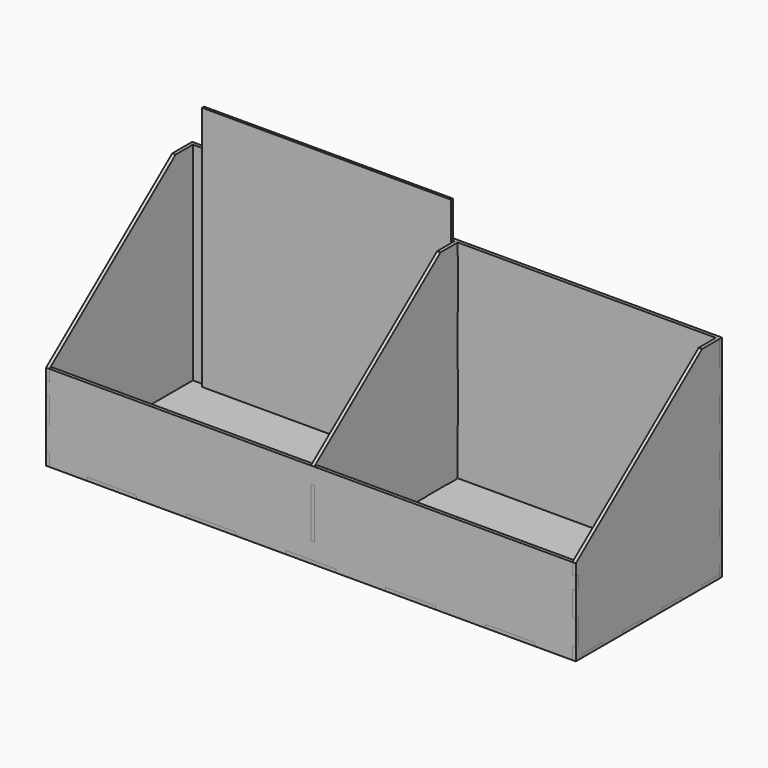
from build123d import *

# Parameters (mm, degrees)
F0_W          = 638
F0_H          = 220
F1_DEPTH      = 4
F2_W          = 638
F2_H          = 4
F3_DEPTH      = 100
F3_DEPTH_BACK = 4
F4_W          = 638
F4_H          = 4
F5_DEPTH      = 250
F5_DEPTH_BACK = 4
F7_DEPTH      = 4
F10_W         = 3
F10_H         = 300
F11_DEPTH     = 300
F12_W         = 4
F12_H         = 30
F12_W_2       = 30
F12_H_2       = 4
F12_H_3       = 15
F13_DEPTH     = 4
F15_W         = 4
F15_H         = 13.8488392308
F15_H_2       = 30
F15_H_3       = 15.1511607692
F15_W_2       = 60
F15_H_4       = 4
F15_W_3       = 4.3
F15_H_5       = 60
F16_DEPTH     = 25
F17_W         = 4
F17_H         = 20
F17_H_2       = 31.2709829547
F17_W_2       = 60
F17_H_3       = 4
F17_W_3       = 30
F17_H_4       = 60
F18_DEPTH     = 25
F19_W         = 4.3
F19_H         = 60
F19_W_2       = 4
F19_H_2       = 30
F19_W_3       = 60
F19_H_3       = 4
F20_DEPTH     = 25
F21_W         = 4.3
F21_H         = 30
F21_W_2       = 60
F21_H_2       = 4
F21_H_3       = 16
F21_W_3       = 4
F22_DEPTH     = 25


with BuildPart() as f1:
    # F0 (on Top) → F1 (new body)
    with BuildSketch(Plane.XY):
        Rectangle(F0_W, F0_H)
    extrude(amount=F1_DEPTH)

    # F21 (on face) → F22 (cut)
    with BuildSketch(Plane(origin=(0, 0, 0), x_dir=(1, 0, 0), z_dir=(0, 0, -1))):
        with Locations((2.15, 45)):
            Rectangle(F21_W, F21_H)
        with Locations((60, 108)):
            Rectangle(F21_W_2, F21_H_2)
        with Locations((180, 108)):
            Rectangle(F21_W_2, F21_H_2)
        Polygon((319, 110), (270, 110), (270, 106), (315, 106), (315, 100), (319, 100), (319, 106), align=None)
        with Locations((2.15, 98)):
            Rectangle(F21_W, F21_H_3)
        with Locations((317, 55)):
            Rectangle(F21_W_3, F21_H)
        with Locations((317, -5)):
            Rectangle(F21_W_3, F21_H)
        Polygon((319, -110), (319, -106), (315, -106), (270, -106), (270, -110), align=None)
        with Locations((2.15, -45)):
            Rectangle(F21_W, F21_H)
        with Locations((2.15, -98)):
            Rectangle(F21_W, F21_H_3)
        with Locations((60, -108)):
            Rectangle(F21_W_2, F21_H_2)
        with Locations((180, -108)):
            Rectangle(F21_W_2, F21_H_2)
        with Locations((317, -65)):
            Rectangle(F21_W_3, F21_H)
        with Locations((-180, 108)):
            Rectangle(F21_W_2, F21_H_2)
        with Locations((-317, -65)):
            Rectangle(F21_W_3, F21_H)
        Polygon((-319, 110), (-319, 106), (-319, 100), (-315, 100), (-315, 106), (-270, 106), (-270, 110), align=None)
        with Locations((-60, 108)):
            Rectangle(F21_W_2, F21_H_2)
        with Locations((-180, -108)):
            Rectangle(F21_W_2, F21_H_2)
        with Locations((-317, -5)):
            Rectangle(F21_W_3, F21_H)
        with Locations((-317, 55)):
            Rectangle(F21_W_3, F21_H)
        with Locations((-60, -108)):
            Rectangle(F21_W_2, F21_H_2)
        Polygon((-319, -110), (-270, -110), (-270, -106), (-315, -106), (-319, -106), align=None)
    extrude(amount=-F22_DEPTH, mode=Mode.SUBTRACT)


with BuildPart() as f3:
    # F2 (on face) → F3 (new body, two sides)
    with BuildSketch(Plane.XY.offset(4)) as f3_sk:
        with Locations((0, -108)):
            Rectangle(F2_W, F2_H)
    extrude(amount=F3_DEPTH)
    extrude(f3_sk.sketch, amount=-F3_DEPTH_BACK)

    # F15 (on face) → F16 (cut)
    with BuildSketch(Plane.XZ.offset(110)):
        with Locations((-317, 97.0755803846)):
            Rectangle(F15_W, F15_H)
        with Locations((-317, 60.1511607692)):
            Rectangle(F15_W, F15_H_2)
        with Locations((-317, 7.5755803846)):
            Rectangle(F15_W, F15_H_3)
        with Locations((317, 97.0755803846)):
            Rectangle(F15_W, F15_H)
        with Locations((317, 60.1511607692)):
            Rectangle(F15_W, F15_H_2)
        with Locations((317, 7.5755803846)):
            Rectangle(F15_W, F15_H_3)
        with Locations((-240, 2)):
            Rectangle(F15_W_2, F15_H_4)
        with Locations((-120, 2)):
            Rectangle(F15_W_2, F15_H_4)
        with Locations((0, 2)):
            Rectangle(F15_W_2, F15_H_4)
        with Locations((120, 2)):
            Rectangle(F15_W_2, F15_H_4)
        with Locations((240, 2)):
            Rectangle(F15_W_2, F15_H_4)
        with Locations((2.15, 54)):
            Rectangle(F15_W_3, F15_H_5)
    extrude(amount=-F16_DEPTH, mode=Mode.SUBTRACT)


with BuildPart() as f5:
    # F4 (on face) → F5 (new body, two sides)
    with BuildSketch(Plane.XY.offset(4)) as f5_sk:
        with Locations((0, 108)):
            Rectangle(F4_W, F4_H)
    extrude(amount=F5_DEPTH)
    extrude(f5_sk.sketch, amount=-F5_DEPTH_BACK)

    # F19 (on face) → F20 (cut)
    with BuildSketch(Plane(origin=(0, 110, 0), x_dir=(-1, 0, 0), z_dir=(0, 1, 0))):
        with Locations((-2.15, 210)):
            Rectangle(F19_W, F19_H)
        with Locations((-2.15, 90)):
            Rectangle(F19_W, F19_H)
        with Locations((317, 209)):
            Rectangle(F19_W_2, F19_H_2)
        with Locations((317, 149)):
            Rectangle(F19_W_2, F19_H_2)
        with Locations((317, 89)):
            Rectangle(F19_W_2, F19_H_2)
        with Locations((317, 29)):
            Rectangle(F19_W_2, F19_H_2)
        with Locations((-317, 209)):
            Rectangle(F19_W_2, F19_H_2)
        with Locations((-317, 89)):
            Rectangle(F19_W_2, F19_H_2)
        with Locations((-317, 29)):
            Rectangle(F19_W_2, F19_H_2)
        with Locations((-317, 149)):
            Rectangle(F19_W_2, F19_H_2)
        with Locations((0, 2)):
            Rectangle(F19_W_3, F19_H_3)
        with Locations((-120, 2)):
            Rectangle(F19_W_3, F19_H_3)
        with Locations((-240, 2)):
            Rectangle(F19_W_3, F19_H_3)
        with Locations((240, 2)):
            Rectangle(F19_W_3, F19_H_3)
        with Locations((120, 2)):
            Rectangle(F19_W_3, F19_H_3)
    extrude(amount=-F20_DEPTH, mode=Mode.SUBTRACT)


with BuildPart() as f7:
    # F6 (on face) → F7 (new body)
    with BuildSketch(Plane(origin=(-319, 0, 0), x_dir=(0, -1, 0), z_dir=(-1, 0, 0))):
        Polygon((-110, 254), (-110, 0), (110, 0), (110, 104), (-80, 254), align=None)
    extrude(amount=-F7_DEPTH)


with BuildPart() as f9_1:
    # F9: instance of F7
    add(f7.part.mirror(Plane(origin=(-157.5, 7.9870285852, 50.3214028345), x_dir=(0, 1, 0), z_dir=(1, 0, 0))))

    # F17 (on face) → F18 (cut)
    with BuildSketch(Plane.YZ.offset(4)):
        with Locations((-108, 94)):
            Rectangle(F17_W, F17_H)
        with Locations((-108, 8.3645085227)):
            Rectangle(F17_W, F17_H_2)
        with Locations((0, 2)):
            Rectangle(F17_W_2, F17_H_3)
        with Locations((-75, 2)):
            Rectangle(F17_W_3, F17_H_3)
        with Locations((75, 2)):
            Rectangle(F17_W_3, F17_H_3)
        with Locations((108, 30)):
            Rectangle(F17_W, F17_H_4)
        with Locations((108, 150)):
            Rectangle(F17_W, F17_H_4)
        with Locations((108, 270)):
            Rectangle(F17_W, F17_H_4)
    extrude(amount=-F18_DEPTH, mode=Mode.SUBTRACT)


with BuildPart() as f11:
    # F10 (on face) → F11 (new body)
    with BuildSketch(Plane(origin=(0, 0, 0), x_dir=(0, -1, 0), z_dir=(-1, 0, 0))):
        with Locations((-102.5, 150)):
            Rectangle(F10_W, F10_H)
    extrude(amount=F11_DEPTH)


with BuildPart() as f7_1:
    add(f7.part)

    # F12 (on face) → F13 (cut)
    with BuildSketch(Plane(origin=(-319, 0, 0), x_dir=(0, -1, 0), z_dir=(-1, 0, 0))):
        with Locations((-108, 239)):
            Rectangle(F12_W, F12_H)
        with Locations((-108, 179)):
            Rectangle(F12_W, F12_H)
        with Locations((-108, 119)):
            Rectangle(F12_W, F12_H)
        with Locations((-108, 59)):
            Rectangle(F12_W, F12_H)
        Polygon((-106, 14), (-110, 14), (-110, 0), (-80, 0), (-80, 4), (-106, 4), align=None)
        with Locations((-35, 2)):
            Rectangle(F12_W_2, F12_H_2)
        with Locations((25, 2)):
            Rectangle(F12_W_2, F12_H_2)
        with Locations((85, 2)):
            Rectangle(F12_W_2, F12_H_2)
        with Locations((108, 30.1511607692)):
            Rectangle(F12_W, F12_H)
        with Locations((108, 82.6511607692)):
            Rectangle(F12_W, F12_H_3)
    extrude(amount=-F13_DEPTH, mode=Mode.SUBTRACT)


with BuildPart() as f14_1:
    # F14: instance of F7
    add(f7_1.part.mirror(Plane.YZ))


solid = Compound([f1.part, f3.part, f5.part, f9_1.part, f11.part, f7_1.part, f14_1.part])
